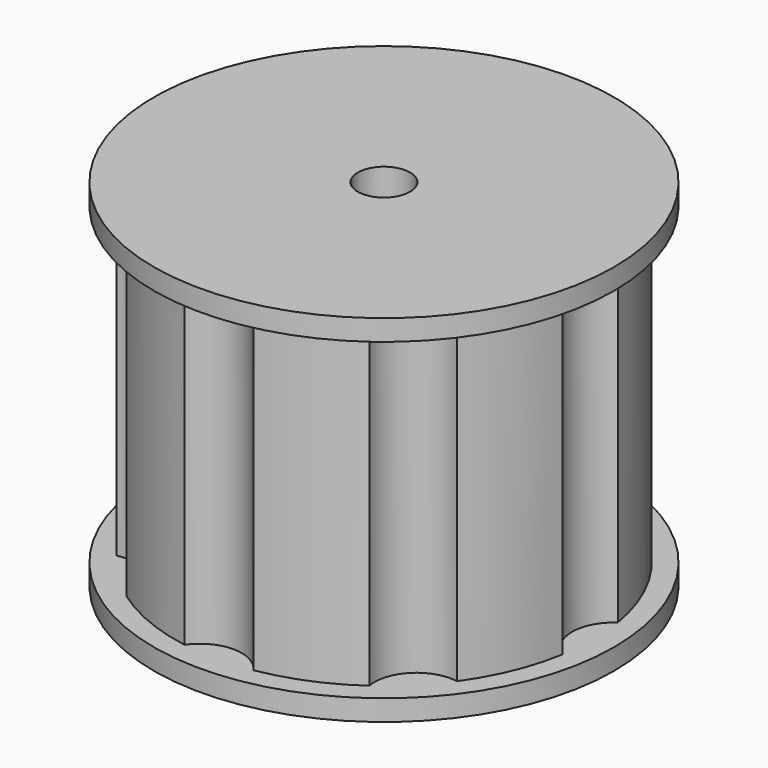
from build123d import *

# Parameters (mm, degrees)
F0_R            = 25.4
F1_DEPTH        = 19.05
F2_R            = 27.94
F2_R_2          = 25.4
F3_DEPTH        = 2.54
F5_DEPTH        = 38.1
F5_COPIES_COUNT = 8
F6_R            = 27.94
F7_DEPTH        = 2.54
F8_R            = 3.175
F9_DEPTH        = 43.181


# Not quite as in the source:
# - a pattern or mirror of a feature is missing from the dataset's text; its kind, count and spacing are read off the source's solid


with BuildPart() as f1:
    # F0 (on Top) → F1 (new body, symmetric)
    with BuildSketch(Plane.XY):
        Circle(F0_R)
    extrude(amount=F1_DEPTH, both=True)

    # F2 (on face) → F3 (join)
    with BuildSketch(Plane.XY.offset(19.05)):
        Circle(F2_R)
        Circle(F2_R_2, mode=Mode.SUBTRACT)
        Circle(F2_R_2)
    extrude(amount=F3_DEPTH)

    # F4 (on face) → F5 (cut, through all)
    with BuildSketch(Plane(origin=(0, 0, -19.05), x_dir=(1, 0, 0), z_dir=(0, 0, -1))):
        with BuildLine():
            ThreePointArc((4.1803474687, 25.0536363636), (0, 25.4), (-4.1803474687, 25.0536363636))
            ThreePointArc((-4.1803474687, 25.0536363636), (0, 22.86), (4.1803474687, 25.0536363636))
        make_face()
    f5 = extrude(amount=-F5_DEPTH, mode=Mode.SUBTRACT)

    # F5_copies: F5 ×8 about axis
    f5_copies_axis = Axis((0, 0, 0), (0, 0, 1))
    for i in range(1, F5_COPIES_COUNT):
        add(f5.rotate(f5_copies_axis, i * 360 / F5_COPIES_COUNT), mode=Mode.SUBTRACT)

    # F6 (on face) → F7 (join)
    with BuildSketch(Plane(origin=(0, 0, -19.05), x_dir=(1, 0, 0), z_dir=(0, 0, -1))):
        Circle(F6_R)
    extrude(amount=F7_DEPTH)

    # F8 (on face) → F9 (cut, through all)
    with BuildSketch(Plane(origin=(0, 0, -21.59), x_dir=(1, 0, 0), z_dir=(0, 0, -1))):
        Circle(F8_R)
    extrude(amount=-F9_DEPTH, mode=Mode.SUBTRACT)


solid = f1.part
